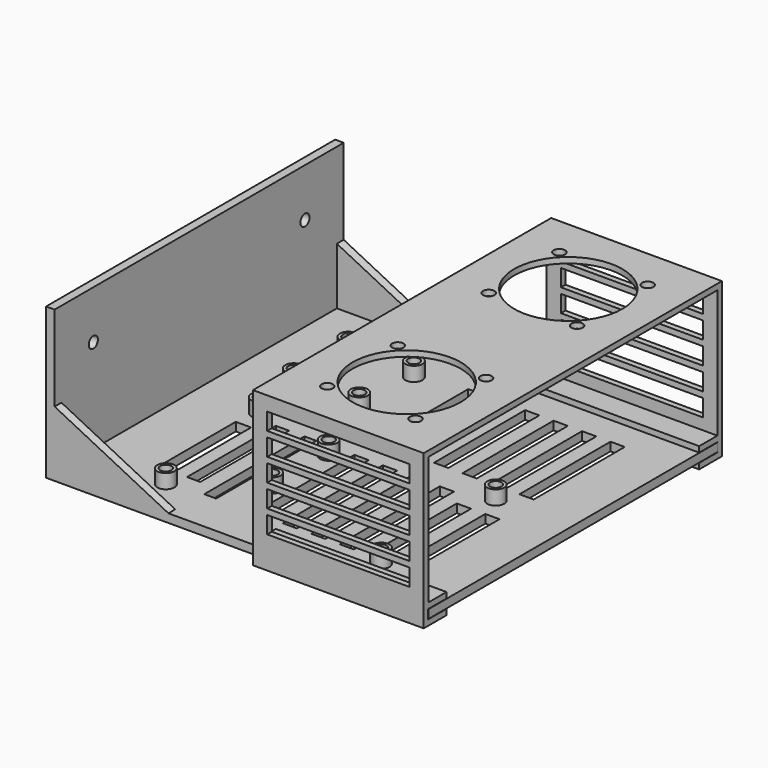
from build123d import *
from build123d import SkipClean  # not in build123d's __all__

# Parameters (mm, degrees)
F0_W      = 134.3
F0_H      = 126.9636089172
F0_R      = 2
F1_DEPTH  = 3
F2_DEPTH  = 25
F3_R      = 3
F3_R_2    = 2
F4_DEPTH  = 5
F5_W      = 3
F5_H      = 126.9636089172
F6_DEPTH  = 50
F7_R      = 2
F8_DEPTH  = 25
F10_DEPTH = 3
F12_DEPTH = 3
F14_DEPTH = 60
F15_R     = 19
F15_R_2   = 2
F16_DEPTH = 25
F17_W     = 50
F17_H     = 6
F18_DEPTH = 200
F19_W     = 5
F19_H     = 34
F19_H_2   = 44
F19_W_2   = 4.1724147481
F19_W_3   = 4.6632857585
F19_H_3   = 39
F19_W_4   = 5.3995953176
F19_H_4   = 40
F20_DEPTH = 25


# Not quite as in the source:
# - after a boolean that leaves OpenCascade's solid faulty, fix() repairs it
# - a feature names something its author has since deleted; it is built from what else it names


with BuildPart() as f1:
    # F0 (on Top) → F1 (new body)
    with BuildSketch(Plane.XY):
        with Locations((-2.35, 26.4818044586)):
            Rectangle(F0_W, F0_H)
        with BuildLine():
            Line((-49.5, 22.5), (-46.5, 27))
            Line((-46.5, 27), (-44.7245493689, 27))
            ThreePointArc((-44.7245493689, 27), (-44.1, 27.1000162933), (-43.4754506311, 27))
            Line((-43.4754506311, 27), (48, 27))
            Line((48, 27), (48, 23.31))
            Line((48, 23.31), (49.6, 23.31))
            Line((49.6, 23.31), (49.6, 14.31))
            Line((49.6, 14.31), (48, 14.31))
            Line((48, 14.31), (48, -5.37))
            Line((48, -5.37), (54.8, -5.37))
            Line((54.8, -5.37), (54.8, -17.5))
            Line((54.8, -17.5), (48, -17.5))
            Line((48, -17.5), (48, -27))
            Line((48, -27), (-46.75, -27))
            Line((-46.75, -27), (-46.75, -14.5))
            Line((-46.75, -14.5), (-49.5, -14.5))
            Line((-49.5, -14.5), (-49.5, 22.5))
        make_face(mode=Mode.SUBTRACT)
        Polygon((-24.5, 70.3), (-22.25, 70.3), (-22.25, 42), (-49.5, 42), (-49.5, 44.3), (-49.5, 68.3), (-49.5, 70.3), (-47.5, 70.3), align=None, mode=Mode.SUBTRACT)
        with BuildLine():
            Line((-44.7245493689, 27), (-46.5, 27))
            Line((-46.5, 27), (-49.5, 22.5))
            Line((-49.5, 22.5), (-49.5, -14.5))
            Line((-49.5, -14.5), (-46.75, -14.5))
            Line((-46.75, -14.5), (-46.75, -27))
            Line((-46.75, -27), (48, -27))
            Line((48, -27), (48, -17.5))
            Line((48, -17.5), (54.8, -17.5))
            Line((54.8, -17.5), (54.8, -5.37))
            Line((54.8, -5.37), (48, -5.37))
            Line((48, -5.37), (48, 14.31))
            Line((48, 14.31), (49.6, 14.31))
            Line((49.6, 14.31), (49.6, 23.31))
            Line((49.6, 23.31), (48, 23.31))
            Line((48, 23.31), (48, 27))
            Line((48, 27), (-43.4754506311, 27))
            ThreePointArc((-43.4754506311, 27), (-42.4799538991, 26.2728123672), (-42.1, 25.1000162933))
            ThreePointArc((-42.1, 25.1000162933), (-45.272796074, 23.4799701924), (-44.7245493689, 27))
        make_face()
        with Locations((-37.82, -24)):
            Circle(F0_R, mode=Mode.SUBTRACT)
        with Locations((-13.4690740741, -7.7952196389)):
            Circle(F0_R, mode=Mode.SUBTRACT)
        with Locations((-13.5170461553, 17.1474736725)):
            Circle(F0_R, mode=Mode.SUBTRACT)
        with Locations((37.78, -24)):
            Circle(F0_R, mode=Mode.SUBTRACT)
        with Locations((38.8999233283, 24.9872000806)):
            Circle(F0_R, mode=Mode.SUBTRACT)
        with BuildLine():
            Line((-22.25, 42), (-22.25, 70.3))
            Line((-22.25, 70.3), (-24.5, 70.3))
            Line((-24.5, 70.3), (-47.5, 70.3))
            ThreePointArc((-47.5, 70.3), (-46.0857864376, 69.7142135624), (-45.5, 68.3))
            ThreePointArc((-45.5, 68.3), (-47.5, 66.3), (-49.5, 68.3))
            Line((-49.5, 68.3), (-49.5, 44.3))
            Line((-49.5, 44.3), (-49.5, 42))
            Line((-49.5, 42), (-22.25, 42))
        make_face()
        with BuildLine():
            ThreePointArc((-45.5, 44.3), (-47.5, 42.3), (-49.5, 44.3))
            ThreePointArc((-49.5, 44.3), (-47.5, 46.3), (-45.5, 44.3))
        make_face(mode=Mode.SUBTRACT)
        with Locations((-24.5, 44.3)):
            Circle(F0_R, mode=Mode.SUBTRACT)
        with BuildLine():
            ThreePointArc((-22.5, 68.3), (-25.9142135624, 66.8857864376), (-24.5, 70.3))
            ThreePointArc((-24.5, 70.3), (-23.0857864376, 69.7142135624), (-22.5, 68.3))
        make_face(mode=Mode.SUBTRACT)
    extrude(amount=F1_DEPTH)

    # F0 (on Top) → F2 (cut)
    with BuildSketch(Plane.XY):
        with BuildLine():
            ThreePointArc((-45.5, 68.3), (-46.0857864376, 69.7142135624), (-47.5, 70.3))
            ThreePointArc((-47.5, 70.3), (-48.9142135624, 69.7142135624), (-49.5, 68.3))
            ThreePointArc((-49.5, 68.3), (-47.5, 66.3), (-45.5, 68.3))
        make_face()
        with BuildLine():
            ThreePointArc((-22.5, 68.3), (-23.0857864376, 69.7142135624), (-24.5, 70.3))
            ThreePointArc((-24.5, 70.3), (-25.9142135624, 66.8857864376), (-22.5, 68.3))
        make_face()
        with BuildLine():
            ThreePointArc((-45.5, 44.3), (-47.5, 46.3), (-49.5, 44.3))
            ThreePointArc((-49.5, 44.3), (-47.5, 42.3), (-45.5, 44.3))
        make_face()
        with Locations((-24.5, 44.3)):
            Circle(F0_R)
        with BuildLine():
            ThreePointArc((-43.4754506311, 27), (-44.1, 27.1000162933), (-44.7245493689, 27))
            Line((-44.7245493689, 27), (-43.4754506311, 27))
        make_face()
        with BuildLine():
            Line((-43.4754506311, 27), (-44.7245493689, 27))
            ThreePointArc((-44.7245493689, 27), (-45.272796074, 23.4799701924), (-42.1, 25.1000162933))
            ThreePointArc((-42.1, 25.1000162933), (-42.4799538991, 26.2728123672), (-43.4754506311, 27))
        make_face()
        with Locations((-13.5170461553, 17.1474736725)):
            Circle(F0_R)
        with Locations((38.8999233283, 24.9872000806)):
            Circle(F0_R)
        with Locations((-13.4690740741, -7.7952196389)):
            Circle(F0_R)
        with Locations((-37.82, -24)):
            Circle(F0_R)
        with Locations((37.78, -24)):
            Circle(F0_R)
    extrude(amount=F2_DEPTH, mode=Mode.SUBTRACT)

    # F3 (on face) → F4 (join)
    with BuildSketch(Plane.XY.offset(3)):
        with Locations((-47.5, 68.3)):
            Circle(F3_R)
        with BuildLine():
            ThreePointArc((-47.5, 70.3), (-46.0857864376, 69.7142135624), (-45.5, 68.3))
            ThreePointArc((-45.5, 68.3), (-47.5, 66.3), (-49.5, 68.3))
            Line((-49.5, 68.3), (-49.5, 70.3))
            Line((-49.5, 70.3), (-47.5, 70.3))
        make_face(mode=Mode.SUBTRACT)
        with Locations((-24.5, 68.3)):
            Circle(F3_R)
        with Locations((-24.5, 68.3)):
            Circle(F3_R_2, mode=Mode.SUBTRACT)
        with Locations((-24.5, 44.3)):
            Circle(F3_R)
        with Locations((-24.5, 44.3)):
            Circle(F3_R_2, mode=Mode.SUBTRACT)
        with Locations((-47.5, 44.3)):
            Circle(F3_R)
        with Locations((-47.5, 44.3)):
            Circle(F3_R_2, mode=Mode.SUBTRACT)
        with Locations((-44.1, 25.1000162933)):
            Circle(F3_R)
        with Locations((-44.1, 25.1000162933)):
            Circle(F3_R_2, mode=Mode.SUBTRACT)
        with Locations((-13.5170461553, 17.1474736725)):
            Circle(F3_R)
        with Locations((-13.5170461553, 17.1474736725)):
            Circle(F3_R_2, mode=Mode.SUBTRACT)
        with Locations((38.8999233283, 24.9872000806)):
            Circle(F3_R)
        with Locations((38.8999233283, 24.9872000806)):
            Circle(F3_R_2, mode=Mode.SUBTRACT)
        with Locations((-13.4690740741, -7.7952196389)):
            Circle(F3_R)
        with Locations((-13.4690740741, -7.7952196389)):
            Circle(F3_R_2, mode=Mode.SUBTRACT)
        with Locations((-37.82, -24)):
            Circle(F3_R)
        with Locations((-37.82, -24)):
            Circle(F3_R_2, mode=Mode.SUBTRACT)
        with Locations((37.78, -24)):
            Circle(F3_R)
        with Locations((37.78, -24)):
            Circle(F3_R_2, mode=Mode.SUBTRACT)
    with SkipClean():  # cleaning this boolean's faces spoils the solid; the shape is the same uncleaned
        extrude(amount=F4_DEPTH)

    # F5 (on face) → F6 (join)
    with BuildSketch(Plane.XY.offset(3)):
        with Locations((-68, 26.4818044586)):
            Rectangle(F5_W, F5_H)
    extrude(amount=F6_DEPTH)

    add(f1.part.fix(), mode=Mode.REPLACE)

    # F7 (on face) → F8 (cut)
    with BuildSketch(Plane.YZ.offset(-66.5)):
        with Locations((-20, 36)):
            Circle(F7_R)
        with Locations((72.9636089172, 36)):
            Circle(F7_R)
    extrude(amount=-F8_DEPTH, mode=Mode.SUBTRACT)

    # F9 (on face) → F10 (join)
    with BuildSketch(Plane.XZ.offset(37)):
        Polygon((-26.5, 3), (-66.5, 23), (-66.5, 3), align=None)
    extrude(amount=-F10_DEPTH)

    # F11 (on face) → F12 (join)
    with BuildSketch(Plane(origin=(0, 89.9636089172, 0), x_dir=(-1, 0, 0), z_dir=(0, 1, 0))):
        Polygon((66.5, 3), (66.5, 23), (26.5, 3), align=None)
    extrude(amount=-F12_DEPTH)

    # F19 (on face) → F20 (cut)
    with BuildSketch(Plane.XY):
        with Locations((44.1262373328, 0)):
            Rectangle(F19_W, F19_H)
        with Locations((24.1262373328, 0)):
            Rectangle(F19_W, F19_H_2)
        with Locations((14.1262373328, 0)):
            Rectangle(F19_W, F19_H_2)
        with Locations((4.1262373328, 0)):
            Rectangle(F19_W, F19_H_2)
        with Locations((-5.8737626672, 0)):
            Rectangle(F19_W, F19_H_2)
        with Locations((-23.837414466, 0)):
            Rectangle(F19_W_2, F19_H_2)
        with Locations((-33.654858008, 2.5)):
            Rectangle(F19_W_3, F19_H_3)
        with Locations((-43.3495822757, 0)):
            Rectangle(F19_W_4, F19_H)
        with Locations((44.1262373328, 52)):
            Rectangle(F19_W, F19_H_4)
        with Locations((24.1262373328, 52)):
            Rectangle(F19_W, F19_H_4)
        with Locations((14.1262373328, 52)):
            Rectangle(F19_W, F19_H_4)
        with Locations((4.1262373328, 52)):
            Rectangle(F19_W, F19_H_4)
        with Locations((-5.8737626672, 52)):
            Rectangle(F19_W, F19_H_4)
        with Locations((34.1262373328, 52)):
            Rectangle(F19_W, F19_H_4)
        with Locations((34.1262373328, 0)):
            Rectangle(F19_W, F19_H)
    extrude(amount=F20_DEPTH, mode=Mode.SUBTRACT)


with BuildPart() as f14:
    # F13 (on face) → F14 (new body)
    with BuildSketch(Plane.YZ.offset(64.8)):
        Polygon((-39, 52.1), (-39, 50.1), (-39, -0.1), (-39, -2.1), (-29, -2.1), (-29, -0.1), (-37.2, -0.1), (-37.2, 3.1), (-29, 3.1), (-29, 5.1), (-37, 5.1), (-37, 50.1), (89.9636089172, 50.1), (89.9636089172, 5.1), (81.9636089172, 5.1), (81.9636089172, 3.1), (90.0636089172, 3.1), (90.0636089172, -0.1), (81.9636089172, -0.1), (81.9636089172, -2.1), (91.9636089172, -2.1), (91.9636089172, 0), (91.9636089172, 50.1), (91.9636089172, 52.1), align=None)
    extrude(amount=-F14_DEPTH)

    # F15 (on face) → F16 (cut)
    with BuildSketch(Plane.XY.offset(52.1)):
        with Locations((34.8, 61.9636089172)):
            Circle(F15_R)
        with Locations((19.3, 77.4636089172)):
            Circle(F15_R_2)
        with Locations((50.3, 77.4636089172)):
            Circle(F15_R_2)
        with Locations((50.3, 46.4636089172)):
            Circle(F15_R_2)
        with Locations((19.3, 46.4636089172)):
            Circle(F15_R_2)
        with Locations((19.3, 6.5)):
            Circle(F15_R_2)
        with Locations((34.8, -9)):
            Circle(F15_R)
        with Locations((50.3, 6.5)):
            Circle(F15_R_2)
        with Locations((19.3, -24.5)):
            Circle(F15_R_2)
        with Locations((50.3, -24.5)):
            Circle(F15_R_2)
    extrude(amount=-F16_DEPTH, mode=Mode.SUBTRACT)

    # F17 (on face) → F18 (cut)
    with BuildSketch(Plane(origin=(0, 91.9636089172, 0), x_dir=(-1, 0, 0), z_dir=(0, 1, 0))):
        with Locations((-34.8, 44.1)):
            Rectangle(F17_W, F17_H)
        with Locations((-34.8, 36.1)):
            Rectangle(F17_W, F17_H)
        with Locations((-34.8, 28.1)):
            Rectangle(F17_W, F17_H)
        with Locations((-34.8, 20.1)):
            Rectangle(F17_W, F17_H)
        with Locations((-34.8, 12.1)):
            Rectangle(F17_W, F17_H)
    extrude(amount=-F18_DEPTH, mode=Mode.SUBTRACT)


solid = Compound([f1.part, f14.part])
